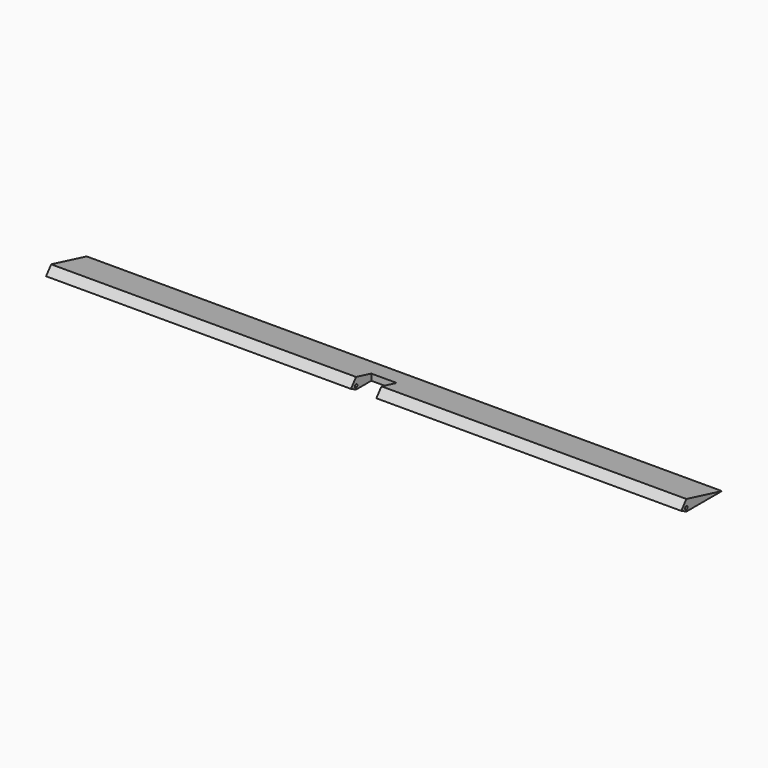
from build123d import *

# Parameters (mm, degrees)
F1_DEPTH   = 762
F2_W       = 12.7
F2_H       = 25.4
F1_FACE1_W = 762
F1_FACE1_H = 7.0995158286
F3_DEPTH   = 38.101
F5_DEPTH   = 635.001
F7_DEPTH   = 635.001


# Not quite as in the source:
# - a feature names something its author has since deleted; it is built from what else it names


with BuildPart() as f1:
    # F0 (on Right) → F1 (new body)
    with BuildSketch(Plane.YZ):
        Polygon((-76.2, 6.35), (-127, -15.875), (-120.65, -19.05), (127, -19.05), (-25.4, 19.05), align=None)
    extrude(amount=F1_DEPTH)

    # F2 (on face) + F1_face1 (on face) → F3 (cut, through all)
    with BuildSketch(Plane(origin=(0, 0, -19.05), x_dir=(1, 0, 0), z_dir=(0, 0, -1))):
        Polygon((0, 120.65), (0, -127), (76.2, -127), (76.2, -76.2), (381, -76.2), (393.7, -76.2), (406.4, -76.2), (711.2, -76.2), (711.2, -127), (762, -127), (762, 120.65), align=None)
        with Locations((387.35, -88.9)):
            Rectangle(F2_W, F2_H)
        with Locations((400.05, -88.9)):
            Rectangle(F2_W, F2_H)
    with BuildSketch(Plane(origin=(381, -123.825, -17.4625), x_dir=(1, 0, 0), z_dir=(0, -0.4472135955, -0.894427191))):
        Rectangle(F1_FACE1_W, F1_FACE1_H)
    extrude(amount=-F3_DEPTH, dir=(0, 0, -1), mode=Mode.SUBTRACT)

    # F4 (on face) → F5 (cut, through all)
    with BuildSketch(Plane(origin=(76.2, 0, 0), x_dir=(0, -1, 0), z_dir=(-1, 0, 0))):
        Polygon((-76.2, -6.35), (-82.55, -7.9375), (-76.2, -15.875), align=None)
        Polygon((-76.2, -15.875), (-82.55, -19.05), (-76.2, -19.05), align=None)
    extrude(amount=-F5_DEPTH, mode=Mode.SUBTRACT)

    # F6 (on face) → F7 (cut, through all)
    with BuildSketch(Plane(origin=(76.2, 0, 0), x_dir=(0, -1, 0), z_dir=(-1, 0, 0))):
        with BuildLine():
            ThreePointArc((-82.55, -17.4625), (-81.4274679849, -16.9975320151), (-80.9625, -15.875))
            ThreePointArc((-80.9625, -15.875), (-83.6725320151, -14.7524679849), (-82.55, -17.4625))
        make_face()
    extrude(amount=-F7_DEPTH, mode=Mode.SUBTRACT)


solid = f1.part
